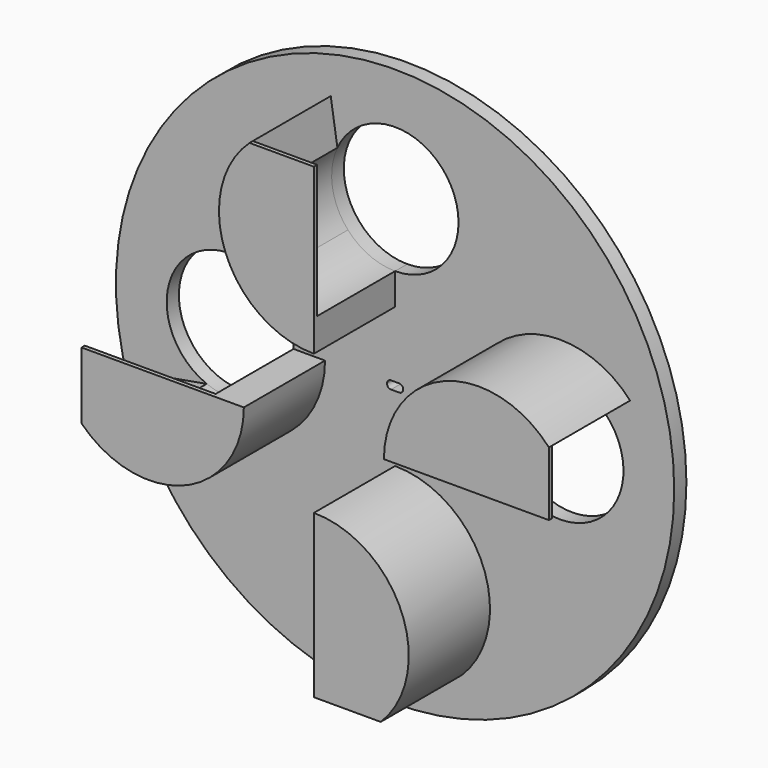
from build123d import *

# Parameters (mm, degrees)
F0_R     = 34.925
F0_R_2   = 7.9375
F1_DEPTH = 1.905
F3_DEPTH = 12.7
F8_DEPTH = 0.508
F9_R     = 0.50799


# Not quite as in the source:
# - a fillet or chamfer is up to 0.001 mm smaller than in the source, because OpenCascade refuses the exact size


with BuildPart() as f1:
    # F0 (on Front) → F1 (new body)
    with BuildSketch(Plane.XZ):
        Circle(F0_R)
        with BuildLine():
            ThreePointArc((7.9375, -20.6375), (-5.6126600757, -26.2501600757), (0, -12.7))
            ThreePointArc((0, -12.7), (5.6126600757, -15.0248399243), (7.9375, -20.6375))
        make_face(mode=Mode.SUBTRACT)
        with Locations((-20.6375, 0)):
            Circle(F0_R_2, mode=Mode.SUBTRACT)
        Polygon((-1.016, 0), (-1.016, 0.508), (0, 0.508), (1.016, 0.508), (1.016, 0), (1.016, -0.508), (0, -0.508), (-1.016, -0.508), align=None, mode=Mode.SUBTRACT)
        with BuildLine():
            ThreePointArc((28.575, 0), (20.6375, -7.9375), (12.7, 0))
            ThreePointArc((12.7, 0), (20.6375, 7.9375), (28.575, 0))
        make_face(mode=Mode.SUBTRACT)
        with BuildLine():
            ThreePointArc((7.9375, 20.6375), (5.6126600757, 15.0248399243), (0, 12.7))
            ThreePointArc((0, 12.7), (-5.6126600757, 26.2501600757), (7.9375, 20.6375))
        make_face(mode=Mode.SUBTRACT)
    extrude(amount=F1_DEPTH)

    # F2 (on face) → F3 (join)
    with BuildSketch(Plane.XZ.offset(1.905)):
        with BuildLine():
            Line((-7.217116123, 23.9416097315), (-8.0497858212, 29.3670302556))
            ThreePointArc((-8.0497858212, 29.3670302556), (-11.0603471299, 16.316334461), (0, 8.763))
            Line((0, 8.763), (0, 12.7))
            ThreePointArc((0, 12.7), (-3.2253143504, 13.384827831), (-5.894084441, 15.3211408274))
            ThreePointArc((-5.894084441, 15.3211408274), (-7.8456367548, 19.4333861511), (-7.217116123, 23.9416097315))
        make_face()
        with BuildLine():
            Line((-23.5666824339, -7.3772485737), (-29.061654765, -8.3688330575))
            ThreePointArc((-29.061654765, -8.3688330575), (-16.1114020949, -10.9780776097), (-8.763, 0))
            Line((-8.763, 0), (-12.7, 0))
            ThreePointArc((-12.7, 0), (-13.3830221995, -3.2212510135), (-15.3145406216, -5.8881244642))
            ThreePointArc((-15.3145406216, -5.8881244642), (-19.2279203931, -7.8113373747), (-23.5666824339, -7.3772485737))
        make_face()
        with BuildLine():
            Line((23.9903295305, 7.1946118999), (29.4060203782, 8.0072967115))
            ThreePointArc((29.4060203782, 8.0072967115), (16.3432040729, 11.0708072308), (8.763, 0))
            Line((8.763, 0), (12.7, 0))
            ThreePointArc((12.7, 0), (13.384689213, 3.225002626), (15.3206341891, 5.8936274228))
            ThreePointArc((15.3206341891, 5.8936274228), (19.4595781944, 7.8496118675), (23.9903295305, 7.1946118999))
        make_face()
        with BuildLine():
            Line((7.374412056, -23.5738162429), (8.3621654342, -29.0682733631))
            ThreePointArc((8.3621654342, -29.0682733631), (10.9798672248, -16.1157452549), (0, -8.763))
            Line((0, -8.763), (0, -12.7))
            ThreePointArc((0, -12.7), (3.2225232211, -13.3835872393), (5.8899911345, -15.3166062137))
            ThreePointArc((5.8899911345, -15.3166062137), (7.4079589254, -17.786877119), (7.9375, -20.6375))
            ThreePointArc((7.9375, -20.6375), (7.7954570727, -22.1324097892), (7.374412056, -23.5738162429))
        make_face()
    extrude(amount=F3_DEPTH)

    # F4 (on face) + F7 (on face) + F6 (on face) + F5 (on face) → F8 (join)
    with BuildSketch(Plane.XZ.offset(14.605)):
        with BuildLine():
            Line((-12.7, 0), (-20.6375, 0))
            Line((-20.6375, 0), (-23.5666824339, 0))
            Line((-23.5666824339, 0), (-23.5666824339, -7.3772485737))
            ThreePointArc((-23.5666824339, -7.3772485737), (-16.1791639494, -6.567126153), (-12.7, 0))
        make_face()
        Polygon((-23.5666824339, -7.3772485737), (-23.5666824339, 0), (-29.061654765, 0), (-29.061654765, -8.3688330575), align=None)
    with BuildSketch(Plane.XZ.offset(14.605)):
        with BuildLine():
            Line((0, 23.9416097315), (-7.217116123, 23.9416097315))
            ThreePointArc((-7.217116123, 23.9416097315), (-6.6794564616, 16.3492873621), (0, 12.7))
            Line((0, 12.7), (0, 20.6375))
            Line((0, 20.6375), (0, 23.9416097315))
        make_face()
        Polygon((-8.0497858212, 29.3670302556), (-7.217116123, 23.9416097315), (0, 23.9416097315), (0, 29.3670302556), align=None)
    with BuildSketch(Plane.XZ.offset(14.605)):
        with BuildLine():
            ThreePointArc((23.9903295305, 7.1946118999), (16.3718920801, 6.6939147981), (12.7, 0))
            Line((12.7, 0), (20.6375, 0))
            Line((20.6375, 0), (23.9903295305, 0))
            Line((23.9903295305, 0), (23.9903295305, 7.1946118999))
        make_face()
        Polygon((29.4060203782, 8.0072967115), (23.9903295305, 7.1946118999), (23.9903295305, 0), (29.4060203782, 0), align=None)
    with BuildSketch(Plane.XZ.offset(14.605)):
        with BuildLine():
            Line((0, -12.7), (0, -20.6375))
            Line((0, -20.6375), (0, -23.5738162429))
            Line((0, -23.5738162429), (7.374412056, -23.5738162429))
            ThreePointArc((7.374412056, -23.5738162429), (6.5692814077, -16.1823402906), (0, -12.7))
        make_face()
        Polygon((7.374412056, -23.5738162429), (0, -23.5738162429), (0, -29.0682733631), (8.3621654342, -29.0682733631), align=None)
    extrude(amount=-F8_DEPTH)

    # F9 (radius 0.508 in the source; OpenCascade refuses exactly that, so slightly less here)
    f9_edges = [f1.edges().sort_by_distance(p)[0] for p in [
        (1.016, -0.9525, 0.508),
        (1.016, -0.9525, -0.508),
        (-1.016, -0.9525, -0.508),
        (-1.016, -0.9525, 0.508),
    ]]
    fillet(f9_edges, radius=F9_R)


solid = f1.part
